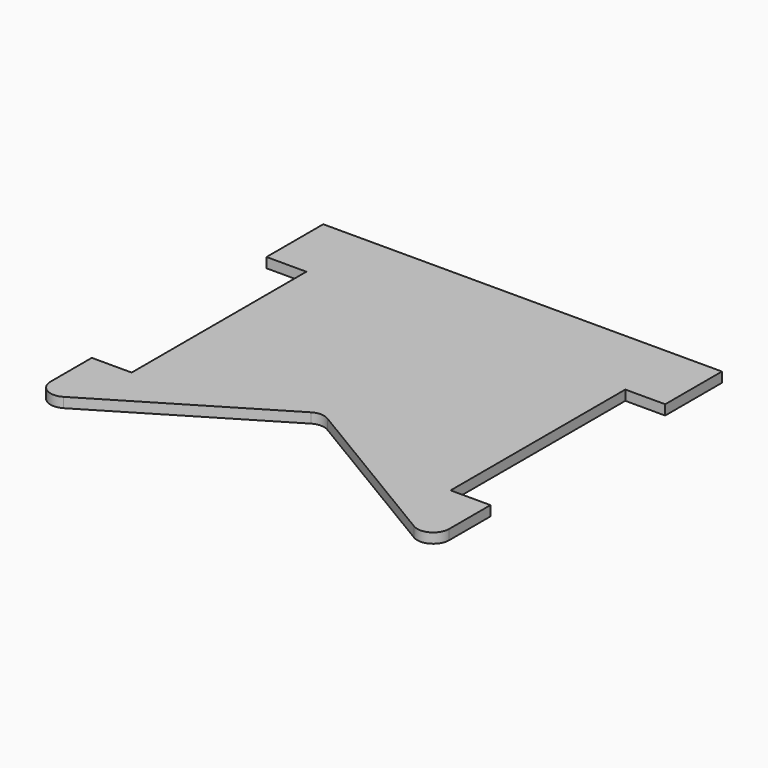
from build123d import *

# Parameters (mm, degrees)
F0_W     = 12.7
F0_H     = 22.5932470911
F1_DEPTH = 3.175
F2_R     = 5.08


# Not quite as in the source:
# - two fillets or chamfers of one size are made in one step
# - a feature names something its author has since deleted; it is built from what else it names


with BuildPart() as f1:
    # F0 (on Top) → F1 (new body)
    with BuildSketch(Plane.XY):
        Polygon((-50.8, 47.1803817213), (-50.8, 24.5871346301), (-50.8, -32.2834653699), (-50.8, -44.9834653699), (-63.5, -44.9834653699), (-63.5, -70.3834653699), (0, -32.2834653699), (63.5, -70.3834653699), (63.5, -44.9834653699), (50.8, -44.9834653699), (50.8, -32.2834653699), (50.8, 24.5871346301), (50.8, 47.1803817213), (0, 47.1803817213), align=None)
        with Locations((-57.15, 35.8837581757)):
            Rectangle(F0_W, F0_H)
        with Locations((57.15, 35.8837581757)):
            Rectangle(F0_W, F0_H)
    extrude(amount=F1_DEPTH)

    # F2
    f2_edges = [f1.edges().sort_by_distance(p)[0] for p in [
        (-63.5, -70.383465, 1.5875),
        (0, -32.283465, 1.5875),
        (63.5, -70.383465, 1.5875),
    ]]
    fillet(f2_edges, radius=F2_R)


solid = f1.part
